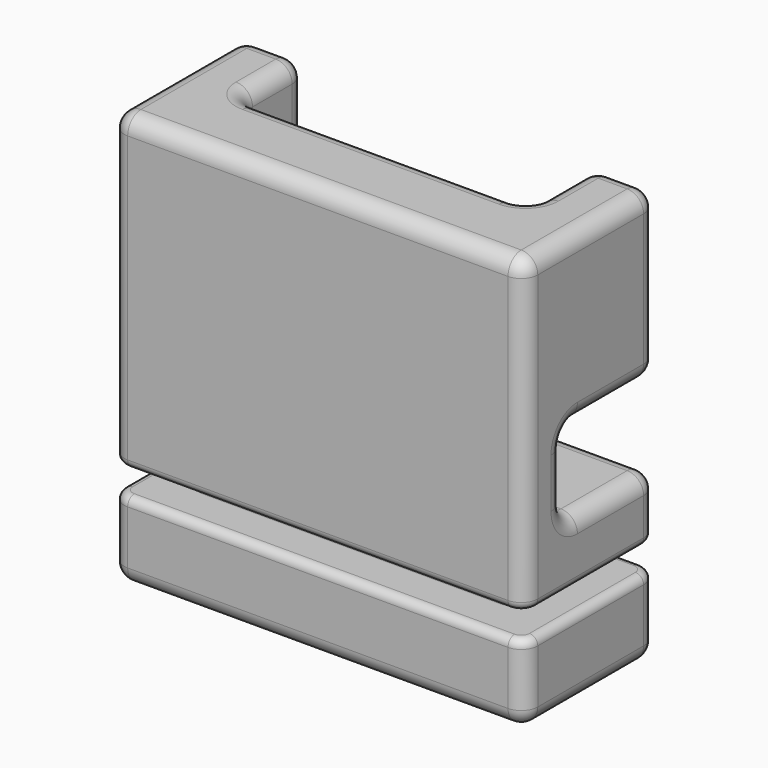
from build123d import *

# Parameters (mm, degrees)
F0_W      = 50
F0_H      = 50
F1_DEPTH  = 10
F2_W      = 14
F2_H      = 10
F3_DEPTH  = 76.70555
F4_F1_R   = 2
F4_F2_R   = 2
F5_W      = 13.7121686712
F5_H      = 20
F6_DEPTH  = 17.5
F7_R      = 2
F8_W      = 3
F8_H      = 5.7575751543
F9_DEPTH  = 29.7216
F10_R     = 1
F11_W     = 46
F11_H     = 3
F11_W_2   = 2
F12_DEPTH = 6
F13_W     = 7.5689357519
F13_H     = 3
F13_W_2   = 12
F14_DEPTH = 6
F15_W     = 8.5923536867
F15_H     = 3
F15_W_2   = 42
F16_DEPTH = 6
F17_W     = 8
F17_H     = 3
F18_DEPTH = 6
F19_R     = 1


with BuildPart() as f1:
    # F0 (on Front) → F1 (new body, symmetric)
    with BuildSketch(Plane.XZ):
        Rectangle(F0_W, F0_H)
    extrude(amount=F1_DEPTH, both=True)

    # F2 (on face) → F3 (cut)
    with BuildSketch(Plane.YZ.offset(25)):
        with Locations((3, 0)):
            Rectangle(F2_W, F2_H)
    extrude(amount=-F3_DEPTH, mode=Mode.SUBTRACT)

    # F4: fillet of radius 2 on 20 edges, made by hand

    # F4_f1
    f4_f1_edges = [f1.edges().sort_by_distance(p)[0] for p in [
        (0, -4, -5),
        (0, -4, 5),
    ]]
    fillet(f4_f1_edges, radius=F4_F1_R)

    # F4_f2
    f4_f2_edges = [f1.edges().sort_by_distance(p)[0] for p in [
        (0, 10, 25),
        (0, -10, 25),
        (0, 10, -5),
        (0, 10, -25),
        (0, -10, -25),
        (25, -10, 0),
        (25, 10, -15),
        (-25, 10, -15),
        (-25, -10, 0),
        (-25, 10, 15),
        (-25, 0, 25),
        (25, 0, 25),
        (25, 10, 15),
        (25, 4, -5),
        (0, 10, 5),
        (-25, 4, 5),
        (-25, 0, -25),
        (25, 0, -25),
        (-25, -3.4142135624, 4.4142135624),
        (25, -3.4142135624, -4.4142135624),
    ]]
    fillet(f4_f2_edges, radius=F4_F2_R)

    # F5 (on Right) → F6 (cut, symmetric)
    with BuildSketch(Plane.YZ):
        with Locations((6.8560843356, 20)):
            Rectangle(F5_W, F5_H)
    extrude(amount=F6_DEPTH, both=True, mode=Mode.SUBTRACT)

    # F7
    f7_edges = [f1.edges().sort_by_distance(p)[0] for p in [
        (0, 0, 10),
        (0, 0, 25),
        (17.5, 4, 25),
        (17.5, 5, 10),
        (0, 10, 10),
        (-17.5, 5, 10),
        (-17.5, 0, 17.5),
        (17.5, 0, 17.5),
        (-17.5, 10, 16.5),
        (17.5, 10, 16.5),
        (-17.5, 9.414214, 24.414214),
        (17.5, 9.414214, 24.414214),
    ]]
    fillet(f7_edges, radius=F7_R)

    # F8 (on Top) → F9 (cut)
    with BuildSketch(Plane.XY):
        with Locations((3.5149400131, 8.914668113)):
            Rectangle(F8_W, F8_H)
        with Locations((-3.5149400131, 8.914668113)):
            Rectangle(F8_W, F8_H)
    extrude(amount=F9_DEPTH, mode=Mode.SUBTRACT)

    # F10
    f10_edges = [f1.edges().sort_by_distance(p)[0] for p in [
        (3.51494, 6.035881, 10),
        (2.01494, 6.035881, 7.5),
        (2.01494, 7.01794, 10),
        (-3.51494, 6.035881, 10),
        (-5.01494, 7.01794, 10),
        (3.51494, 6.035881, 5),
        (5.01494, 6.035881, 7.5),
        (5.01494, 9.414214, 5.585786),
        (-2.01494, 7.01794, 5),
        (-3.51494, 6.035881, 5),
        (-2.01494, 6.035881, 7.5),
        (-5.01494, 6.035881, 7.5),
    ]]
    fillet(f10_edges, radius=F10_R)

    # F11 (on face) → F12 (cut)
    with BuildSketch(Plane(origin=(0, 10, 0), x_dir=(-1, 0, 0), z_dir=(0, 1, 0))):
        with Locations((0, -14)):
            Rectangle(F11_W, F11_H)
        with Locations((-24, -14)):
            Rectangle(F11_W_2, F11_H)
        with Locations((24, -14)):
            Rectangle(F11_W_2, F11_H)
    extrude(amount=-F12_DEPTH, mode=Mode.SUBTRACT)

    # F13 (on face) → F14 (cut)
    with BuildSketch(Plane.YZ.offset(25)):
        with Locations((-11.784467876, -14)):
            Rectangle(F13_W, F13_H)
        with Locations((-2, -14)):
            Rectangle(F13_W_2, F13_H)
    extrude(amount=-F14_DEPTH, mode=Mode.SUBTRACT)

    # F15 (on face) → F16 (cut)
    with BuildSketch(Plane.XZ.offset(10)):
        with Locations((-27.2961768433, -14)):
            Rectangle(F15_W, F15_H)
        with Locations((-2, -14)):
            Rectangle(F15_W_2, F15_H)
    extrude(amount=-F16_DEPTH, mode=Mode.SUBTRACT)

    # F17 (on face) → F18 (cut)
    with BuildSketch(Plane(origin=(-25, 0, 0), x_dir=(0, -1, 0), z_dir=(-1, 0, 0))):
        with Locations((0, -14)):
            Rectangle(F17_W, F17_H)
        Polygon((8, -12.5), (4, -12.5), (4, -15.5), (8, -15.5), (13.1623027846, -15.5), (13.1623027846, -12.5), align=None)
    extrude(amount=-F18_DEPTH, mode=Mode.SUBTRACT)

    # F19
    f19_edges = [f1.edges().sort_by_distance(p)[0] for p in [
        (0, 10, -15.5),
        (0, 4, -15.5),
        (19, 0, -12.5),
        (0, 4, -12.5),
        (0, 10, -12.5),
        (24.414214, 9.414214, -12.5),
        (25, 0, -12.5),
        (19, 4, -14),
        (19, 0, -15.5),
        (25, 0, -15.5),
        (24.414214, 9.414214, -15.5),
        (24.414214, -9.414214, -15.5),
        (0, -4, -15.5),
        (0, -10, -15.5),
        (0, -4, -12.5),
        (0, -10, -12.5),
        (-19, 0, -12.5),
        (-25, 0, -12.5),
        (-24.414214, -9.414214, -12.5),
        (-19, -4, -14),
        (-19, 4, -14),
        (-19, 0, -15.5),
        (-24.414214, 9.414214, -15.5),
        (-25, 0, -15.5),
        (-24.414214, -9.414214, -15.5),
        (-24.414214, 9.414214, -12.5),
        (19, -4, -14),
        (24.414214, -9.414214, -12.5),
    ]]
    fillet(f19_edges, radius=F19_R)


solid = f1.part
